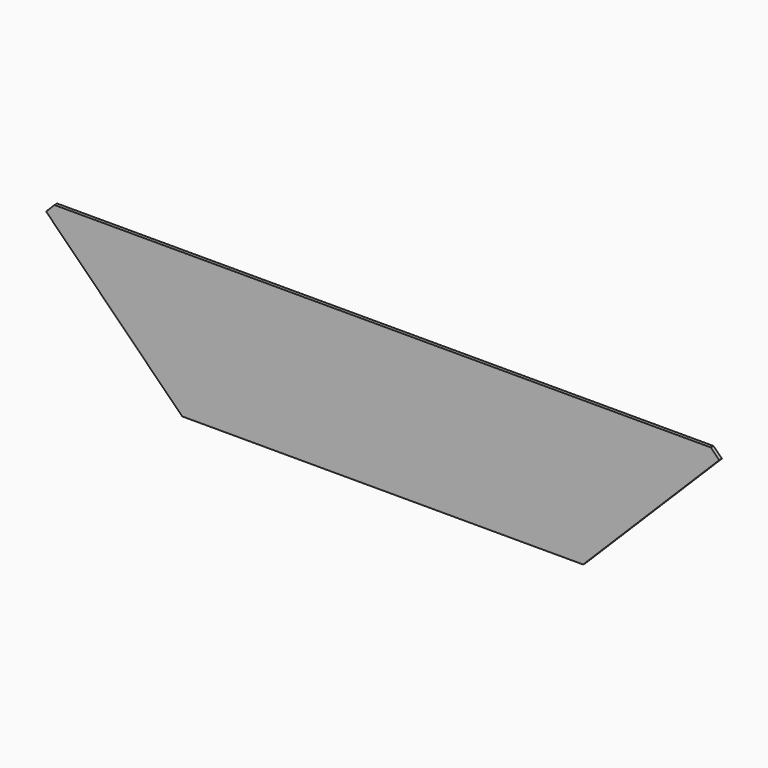
from build123d import *

# Parameters (mm, degrees)
F1_DEPTH = 3.175


# Not quite as in the source:
# - a length typed as a fraction of an inch, garbled in the dataset ("3 / 203.2 mm" for 3/8 in), is restored


with BuildPart() as f1:
    # F0 (on Front) → F1 (new body)
    with BuildSketch(Plane.XZ):
        Polygon((-193.675, 0), (0, 0), (0, 139.7), (-317.1003863096, 139.7), (-325.2376931548, 131.5626931548), align=None)
        Polygon((0, 139.7), (0, 0), (193.675, 0), (325.2376931548, 131.5626931548), (317.1003863096, 139.7), align=None)
    extrude(amount=F1_DEPTH)


solid = f1.part
